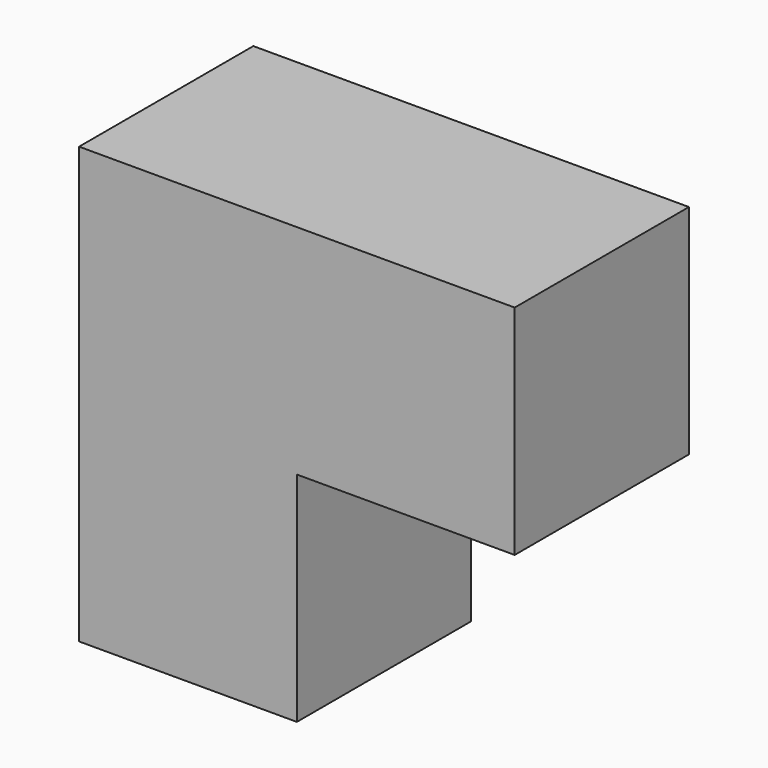
from build123d import *

# Parameters (mm, degrees)
F1_W     = 152.4
F1_H     = 152.4
F2_DEPTH = 76.2
F3_W     = 76.2
F3_H     = 76.2
F4_DEPTH = 76.201


# Not quite as in the source:
# - a variable given as a bare number and used for a length is read in inches; the dataset says mm whatever the document's units were


with BuildPart() as f2:
    # F1 (on Front) → F2 (new body)
    with BuildSketch(Plane.XZ):
        Rectangle(F1_W, F1_H)
    extrude(amount=F2_DEPTH)

    # F3 (on face) → F4 (cut, through all)
    with BuildSketch(Plane.XZ.offset(76.2)):
        with Locations((38.1, -38.1)):
            Rectangle(F3_W, F3_H)
    extrude(amount=-F4_DEPTH, mode=Mode.SUBTRACT)


solid = f2.part
